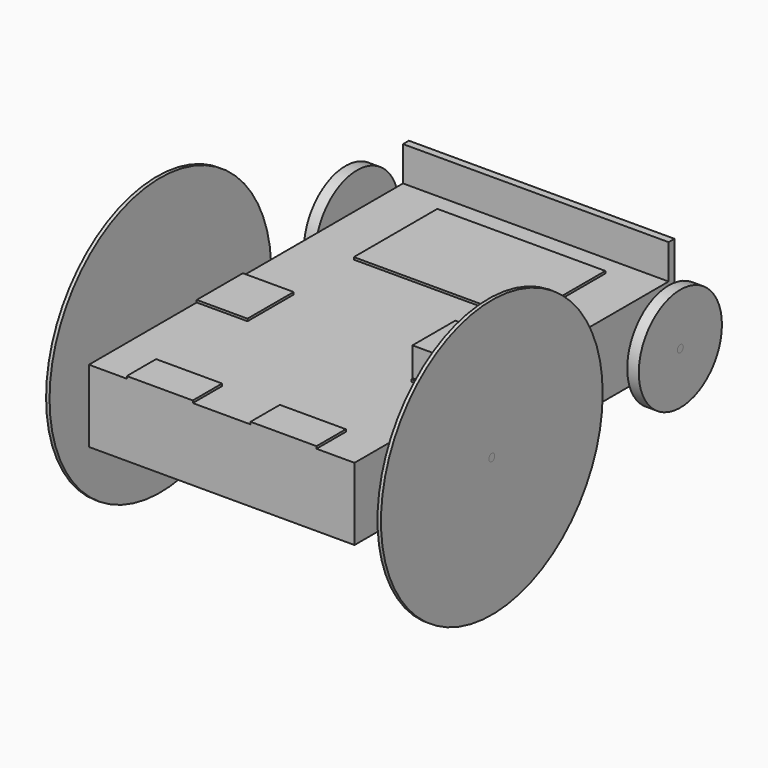
from build123d import *

# Parameters (mm, degrees)
F0_W      = 115
F0_H      = 170
F1_DEPTH  = 3.175
F2_W      = 3.175
F2_H      = 170
F3_DEPTH  = 25
F4_W      = 115
F4_H      = 170
F5_DEPTH  = 3.175
F6_W      = 115
F6_H      = 31.35
F7_DEPTH  = 3.175
F8_W      = 115
F8_H      = 3.175
F9_DEPTH  = 15
F10_R     = 1.5875
F11_DEPTH = 115.001
F12_R     = 1.5875
F13_DEPTH = 15
F14_R     = 1.5875
F15_DEPTH = 15
F16_R     = 1.5875
F17_DEPTH = 15
F18_R     = 1.5875
F19_DEPTH = 15
F20_R     = 1.5875
F21_DEPTH = 15
F22_R     = 1.5875
F23_DEPTH = 15
F24_R     = 1.5875
F25_DEPTH = 15
F26_R     = 1.5875
F27_DEPTH = 15
F28_R     = 60
F28_R_2   = 1.5875
F29_DEPTH = 1.5
F30_R     = 60
F30_R_2   = 1.5875
F31_DEPTH = 1.5
F32_R     = 22.5
F32_R_2   = 1.5875
F33_DEPTH = 5
F34_R     = 22.5
F34_R_2   = 1.5875
F35_DEPTH = 5
F36_R     = 20
F36_R_2   = 1.5875
F37_DEPTH = 6
F38_W     = 22
F38_H     = 25
F39_DEPTH = 1
F40_W     = 22
F40_H     = 23.2
F41_DEPTH = 12.5
F42_R     = 1.5875
F43_DEPTH = 6
F44_R     = 5
F44_R_2   = 1.5875
F45_DEPTH = 6
F46_W     = 72.7409441024
F46_H     = 45.1922491193
F47_DEPTH = 1
F48_W     = 28.58
F48_H     = 15.88
F49_DEPTH = 1


# Not quite as in the source:
# - a length typed as a fraction of an inch, garbled in the dataset ("3 / 203.2 mm" for 3/8 in), is restored


with BuildPart() as f1:
    # F0 (on Top) → F1 (new body)
    with BuildSketch(Plane.XY):
        with Locations((-47.1433209129, 7.6686888933)):
            Rectangle(F0_W, F0_H)
    extrude(amount=F1_DEPTH)

    # F2 (on face) → F3 (join)
    with BuildSketch(Plane(origin=(0, 0, 0), x_dir=(1, 0, 0), z_dir=(0, 0, -1))):
        with Locations((-103.0558209129, -7.6686888933)):
            Rectangle(F2_W, F2_H)
        with Locations((8.7691790871, -7.6686888933)):
            Rectangle(F2_W, F2_H)
    extrude(amount=F3_DEPTH)

    # F4 (on face) → F5 (join)
    with BuildSketch(Plane(origin=(0, 0, -25), x_dir=(1, 0, 0), z_dir=(0, 0, -1))):
        with Locations((-47.1433209129, -7.6686888933)):
            Rectangle(F4_W, F4_H)
    extrude(amount=F5_DEPTH)

    # F6 (on face) → F7 (join)
    with BuildSketch(Plane.XZ.offset(77.3313111067)):
        with Locations((-47.1433209129, -12.5)):
            Rectangle(F6_W, F6_H)
    extrude(amount=F7_DEPTH)

    # F8 (on face) → F9 (join)
    with BuildSketch(Plane.XY.offset(3.175)):
        with Locations((-47.1433209129, 91.0811888933)):
            Rectangle(F8_W, F8_H)
    extrude(amount=F9_DEPTH)

    # F10 (on face) → F11 (cut, through all)
    with BuildSketch(Plane.YZ.offset(10.3566790871)):
        with Locations((-24.9435301409, -12.5)):
            Circle(F10_R)
        with Locations((77.0988376136, -12.5)):
            Circle(F10_R)
    extrude(amount=-F11_DEPTH, mode=Mode.SUBTRACT)

    # F38 (on face) → F39 (join)
    with BuildSketch(Plane.XY.offset(3.175)):
        with Locations((-0.6433209129, -9.6798711922)):
            Rectangle(F38_W, F38_H)
        with Locations((-93.6433209129, -9.6798711922)):
            Rectangle(F38_W, F38_H)
    extrude(amount=F39_DEPTH)

    # F46 (on face) → F47 (join)
    with BuildSketch(Plane.XY.offset(3.175)):
        with Locations((-46.3694771752, 58.0915473402)):
            Rectangle(F46_W, F46_H)
    extrude(amount=F47_DEPTH)

    # F48 (on face) → F49 (join)
    with BuildSketch(Plane.XY.offset(3.175)):
        with Locations((-73.9702930069, -72.5663111067)):
            Rectangle(F48_W, F48_H)
        with Locations((-20.3902930069, -72.5663111067)):
            Rectangle(F48_W, F48_H)
    extrude(amount=F49_DEPTH)


with BuildPart() as f13:
    # F12 (on face) → F13 (new body)
    with BuildSketch(Plane.YZ.offset(10.3566790871)):
        with Locations((-24.9435301409, -12.5)):
            Circle(F12_R)
    extrude(amount=-F13_DEPTH)

    # F14 (on face) → F15 (join)
    with BuildSketch(Plane.YZ.offset(10.3566790871)):
        with Locations((-24.9435301409, -12.5)):
            Circle(F14_R)
    extrude(amount=F15_DEPTH)


with BuildPart() as f17:
    # F16 (on face) → F17 (new body)
    with BuildSketch(Plane.YZ.offset(10.3566790871)):
        with Locations((77.0988376136, -12.5)):
            Circle(F16_R)
    extrude(amount=-F17_DEPTH)

    # F18 (on face) → F19 (join)
    with BuildSketch(Plane.YZ.offset(10.3566790871)):
        with Locations((77.0988376136, -12.5)):
            Circle(F18_R)
    extrude(amount=F19_DEPTH)


with BuildPart() as f21:
    # F20 (on face) → F21 (new body)
    with BuildSketch(Plane(origin=(-104.6433209129, 0, 0), x_dir=(0, -1, 0), z_dir=(-1, 0, 0))):
        with Locations((24.9435301409, -12.5)):
            Circle(F20_R)
    extrude(amount=-F21_DEPTH)

    # F22 (on face) → F23 (join)
    with BuildSketch(Plane(origin=(-104.6433209129, 0, 0), x_dir=(0, -1, 0), z_dir=(-1, 0, 0))):
        with Locations((24.9435301409, -12.5)):
            Circle(F22_R)
    extrude(amount=F23_DEPTH)


with BuildPart() as f25:
    # F24 (on face) → F25 (new body)
    with BuildSketch(Plane(origin=(-104.6433209129, 0, 0), x_dir=(0, -1, 0), z_dir=(-1, 0, 0))):
        with Locations((-77.0988376136, -12.5)):
            Circle(F24_R)
    extrude(amount=-F25_DEPTH)

    # F26 (on face) → F27 (join)
    with BuildSketch(Plane(origin=(-104.6433209129, 0, 0), x_dir=(0, -1, 0), z_dir=(-1, 0, 0))):
        with Locations((-77.0988376136, -12.5)):
            Circle(F26_R)
    extrude(amount=F27_DEPTH)


with BuildPart() as f29:
    # F28 (on face) → F29 (new body)
    with BuildSketch(Plane(origin=(-119.6433209129, 0, 0), x_dir=(0, -1, 0), z_dir=(-1, 0, 0))):
        with Locations((24.9435301409, -12.5)):
            Circle(F28_R)
        with Locations((24.9435301409, -12.5)):
            Circle(F28_R_2, mode=Mode.SUBTRACT)
    extrude(amount=-F29_DEPTH)


with BuildPart() as f31:
    # F30 (on face) → F31 (new body)
    with BuildSketch(Plane.YZ.offset(25.3566790871)):
        with Locations((-24.9435301409, -12.5)):
            Circle(F30_R)
        with Locations((-24.9435301409, -12.5)):
            Circle(F30_R_2, mode=Mode.SUBTRACT)
    extrude(amount=-F31_DEPTH)


with BuildPart() as f33:
    # F32 (on face) → F33 (new body)
    with BuildSketch(Plane.YZ.offset(25.3566790871)):
        with Locations((77.0988376136, -12.5)):
            Circle(F32_R)
        with Locations((77.0988376136, -12.5)):
            Circle(F32_R_2, mode=Mode.SUBTRACT)
    extrude(amount=-F33_DEPTH)


with BuildPart() as f35:
    # F34 (on face) → F35 (new body)
    with BuildSketch(Plane(origin=(-119.6433209129, 0, 0), x_dir=(0, -1, 0), z_dir=(-1, 0, 0))):
        with Locations((-77.0988376136, -12.5)):
            Circle(F34_R)
        with Locations((-77.0988376136, -12.5)):
            Circle(F34_R_2, mode=Mode.SUBTRACT)
    extrude(amount=-F35_DEPTH)


with BuildPart() as f37:
    # F36 (on face) → F37 (new body)
    with BuildSketch(Plane(origin=(23.8566790871, 0, 0), x_dir=(0, -1, 0), z_dir=(-1, 0, 0))):
        with Locations((24.9435301409, -12.5)):
            Circle(F36_R)
        with Locations((24.9435301409, -12.5)):
            Circle(F36_R_2, mode=Mode.SUBTRACT)
    extrude(amount=F37_DEPTH)


with BuildPart() as f41:
    # F40 (on face) → F41 (new body)
    with BuildSketch(Plane.XY.offset(4.175)):
        with Locations((-0.881407346, -9.7505884518)):
            Rectangle(F40_W, F40_H)
    extrude(amount=F41_DEPTH)

    # F42 (on face) → F43 (join)
    with BuildSketch(Plane.YZ.offset(10.118592654)):
        with Locations((-15.1921858778, 10.4964692146)):
            Circle(F42_R)
    extrude(amount=F43_DEPTH)


with BuildPart() as f45:
    # F44 (on face) → F45 (new body)
    with BuildSketch(Plane.YZ.offset(16.118592654)):
        with Locations((-15.1921858778, 10.4964692146)):
            Circle(F44_R)
        with Locations((-15.1921858778, 10.4964692146)):
            Circle(F44_R_2, mode=Mode.SUBTRACT)
    extrude(amount=-F45_DEPTH)


solid = Compound([f1.part, f13.part, f17.part, f21.part, f25.part, f29.part, f31.part, f33.part, f35.part, f37.part, f41.part, f45.part])
